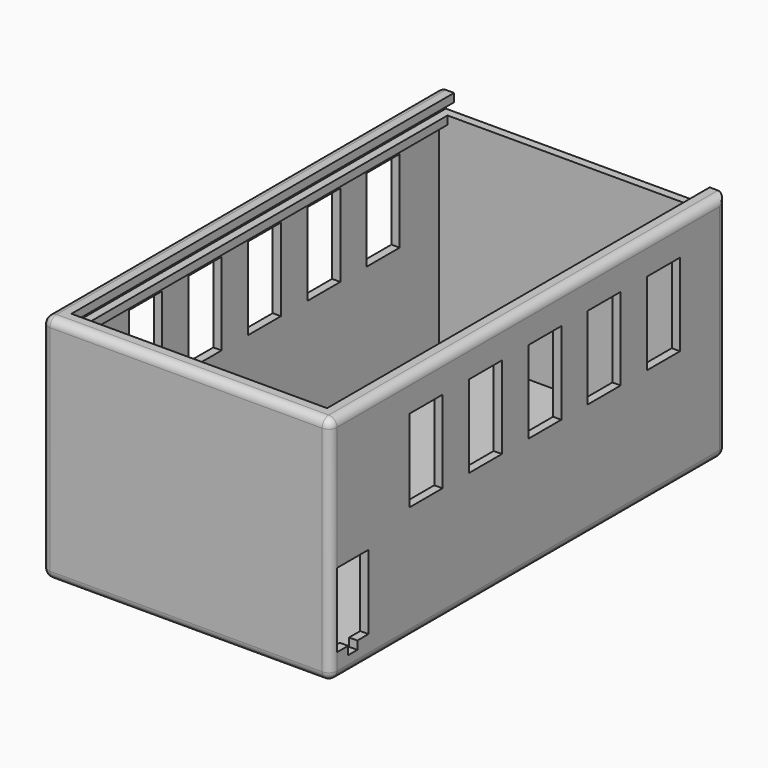
from build123d import *

# Parameters (mm, degrees)
F0_W      = 152.4
F0_H      = 71.12
F1_DEPTH  = 44.45
F2_T      = -2.54
F3_W      = 2.54
F3_H      = 63.5
F4_DEPTH  = 83.82
F5_W      = 147.32
F5_H      = 2.54
F5_W_2    = 149.86
F6_DEPTH  = 2.54
F7_W      = 147.32
F7_H      = 2.54
F7_W_2    = 149.86
F8_DEPTH  = 2.54
F9_W      = 78.74
F9_H      = 2.54
F10_DEPTH = 2.54
F11_W     = 3.556
F11_H     = 2.54
F12_DEPTH = 127
F13_R     = 2.53999
F14_W     = 12.7
F14_H     = 25.4
F15_DEPTH = 254


# Not quite as in the source:
# - a fillet or chamfer is up to 0.001 mm smaller than in the source, because OpenCascade refuses the exact size


with BuildPart() as f1:
    # F0 (on Right) → F1 (new body, symmetric)
    with BuildSketch(Plane.YZ):
        Rectangle(F0_W, F0_H)
    extrude(amount=F1_DEPTH, both=True)

    # F2
    f2_openings = [f1.faces().sort_by_distance(p)[0] for p in [
        (0, 0, 35.56),
        (0, 76.2, 0),
    ]]
    offset(amount=F2_T, openings=f2_openings)

    # F3 (on face) → F4 (join, through all)
    with BuildSketch(Plane.YZ.offset(-41.91)):
        with Locations((74.93, -1.27)):
            Rectangle(F3_W, F3_H)
    extrude(amount=F4_DEPTH)

    # F5 (on face) → F6 (join)
    with BuildSketch(Plane(origin=(41.91, 0, 0), x_dir=(0, -1, 0), z_dir=(-1, 0, 0))):
        with Locations((0, 29.21)):
            Rectangle(F5_W, F5_H)
        with Locations((-1.27, 34.29)):
            Rectangle(F5_W_2, F5_H)
    extrude(amount=F6_DEPTH)

    # F7 (on face) → F8 (join)
    with BuildSketch(Plane.YZ.offset(-41.91)):
        with Locations((0, 29.21)):
            Rectangle(F7_W, F7_H)
        with Locations((1.27, 34.29)):
            Rectangle(F7_W_2, F7_H)
    extrude(amount=F8_DEPTH)

    # F9 (on face) → F10 (join)
    with BuildSketch(Plane(origin=(0, -73.66, 0), x_dir=(-1, 0, 0), z_dir=(0, 1, 0))):
        with Locations((0, 34.29)):
            Rectangle(F9_W, F9_H)
        with Locations((0, 29.21)):
            Rectangle(F9_W, F9_H)
    extrude(amount=F10_DEPTH)

    # F11 (on face) → F12 (cut, symmetric)
    with BuildSketch(Plane.YZ.offset(-41.91)):
        Polygon((-73.66, -5.08), (-73.66, -27.94), (-69.3801, -27.94), (-69.3801, -25.4), (-65.8241, -25.4), (-65.8241, -27.94), (-61.5442, -27.94), (-61.5442, -5.08), align=None)
        with Locations((-67.6021, -26.67)):
            Rectangle(F11_W, F11_H)
        with Locations((-67.6021, -29.21)):
            Rectangle(F11_W, F11_H)
    extrude(amount=F12_DEPTH, both=True, mode=Mode.SUBTRACT)

    # F13 (radius 2.54 in the source; OpenCascade refuses exactly that, so slightly less here)
    f13_edges = [f1.edges().sort_by_distance(p)[0] for p in [
        (0, -76.2, -35.56),
        (-44.45, 0, -35.56),
        (44.45, 0, -35.56),
        (44.45, -76.2, 0),
        (-44.45, -76.2, 0),
        (0, 76.2, -35.56),
        (44.45, 76.2, 0),
        (-44.45, 76.2, 0),
        (0, -76.2, 35.56),
        (44.45, 0, 35.56),
        (-44.45, 0, 35.56),
    ]]
    fillet(f13_edges, radius=F13_R)

    # F14 (on face) → F15 (cut)
    with BuildSketch(Plane.YZ.offset(44.45)):
        with Locations((-39.37, 12.7)):
            Rectangle(F14_W, F14_H)
        with Locations((-16.51, 12.7)):
            Rectangle(F14_W, F14_H)
        with Locations((6.35, 12.7)):
            Rectangle(F14_W, F14_H)
        with Locations((29.21, 12.7)):
            Rectangle(F14_W, F14_H)
        with Locations((52.07, 12.7)):
            Rectangle(F14_W, F14_H)
    extrude(amount=-F15_DEPTH, mode=Mode.SUBTRACT)


solid = f1.part
